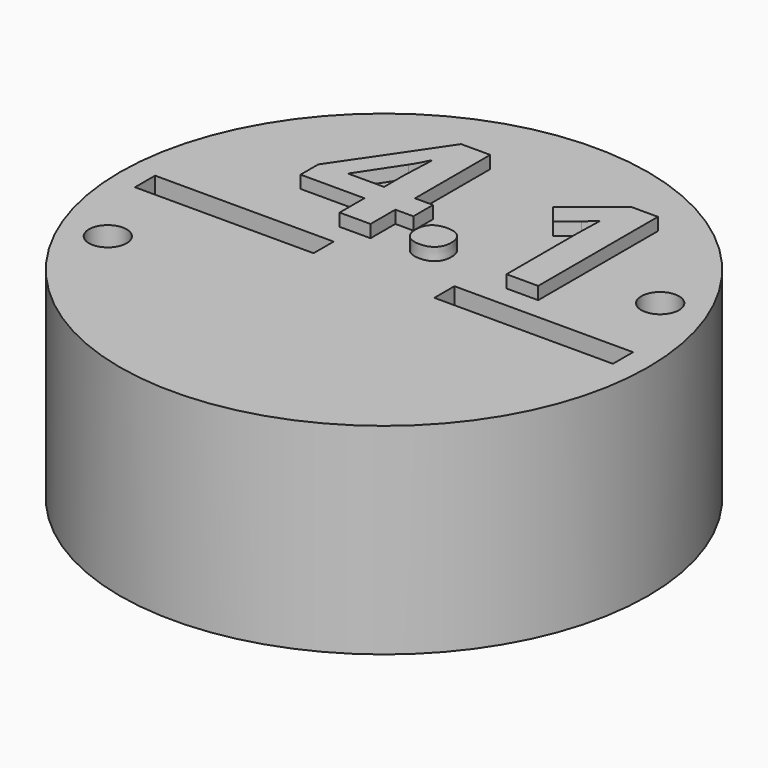
from build123d import *

# Parameters (mm, degrees)
F0_R          = 10.5
F1_DEPTH      = 8
F2_W          = 17.5
F2_H          = 1
F3_DEPTH      = 7
F5_DEPTH      = 17.5
F6_W          = 19
F6_H          = 1
F7_DEPTH      = 7
F9_DEPTH      = 19
F11_DEPTH     = 6.5
F12_R         = 0.75
F12_W         = 7.1
F12_H         = 1
F13_DEPTH     = 8
F14_TEXT_SIZE = 8.3333333333
F15_DEPTH     = 0.5


# Not quite as in the source:
# - Text() gives the source's letters only with a copy of the font that has no kerning and outlines rounded to 1/6400 em; it was checked with that copy


with BuildPart() as f1:
    # F0 (on Top) → F1 (new body)
    with BuildSketch(Plane.XY):
        Circle(F0_R)
    extrude(amount=-F1_DEPTH)

    # F2 (on face) → F3 (cut)
    with BuildSketch(Plane(origin=(0, 0, -8), x_dir=(1, 0, 0), z_dir=(0, 0, -1))):
        Rectangle(F2_W, F2_H)
    extrude(amount=-F3_DEPTH, mode=Mode.SUBTRACT)

    # F4 (on face) → F5 (cut)
    with BuildSketch(Plane(origin=(8.75, 0, 0), x_dir=(0, -1, 0), z_dir=(-1, 0, 0))):
        Polygon((-1.9558809371, -8), (1.9558809371, -8), (1.9558809371, -5), (0.5, -1), (-0.5, -1), (-1.9558809371, -5), align=None)
        Polygon((3, -1.5), (1.3, -1.5), (3, -6.1707116131), align=None)
        Polygon((-3, -6.1707116131), (-1.3, -1.5), (-3, -1.5), align=None)
    extrude(amount=F5_DEPTH, mode=Mode.SUBTRACT)

    # F6 (on face) → F7 (cut)
    with BuildSketch(Plane(origin=(0, 0, -8), x_dir=(1, 0, 0), z_dir=(0, 0, -1))):
        Rectangle(F6_W, F6_H)
    extrude(amount=-F7_DEPTH, mode=Mode.SUBTRACT)

    # F8 (on face) → F9 (cut)
    with BuildSketch(Plane(origin=(9.5, 0, 0), x_dir=(0, -1, 0), z_dir=(-1, 0, 0))):
        Polygon((1.0919107028, -8), (0, -5), (-1.0919107028, -8), align=None)
    extrude(amount=F9_DEPTH, mode=Mode.SUBTRACT)

    # F10 (on face) → F11 (cut)
    with BuildSketch(Plane(origin=(0, 0, -8), x_dir=(1, 0, 0), z_dir=(0, 0, -1))):
        with BuildLine():
            ThreePointArc((9.2870878105, 2.8), (0, 9.7), (-9.2870878105, 2.8))
            Line((-9.2870878105, 2.8), (9.2870878105, 2.8))
        make_face()
        with BuildLine():
            Line((9.3321359979, -2.8), (-9.3321359979, -2.8))
            ThreePointArc((-9.3321359979, -2.8), (0, -9.7431392417), (9.3321359979, -2.8))
        make_face()
    extrude(amount=-F11_DEPTH, mode=Mode.SUBTRACT)

    # F12 (on face) → F13 (cut)
    with BuildSketch(Plane(origin=(0, 0, -8), x_dir=(1, 0, 0), z_dir=(0, 0, -1))):
        with Locations((8.1, -3.6)):
            Circle(F12_R)
        with Locations((-8.1, 3.6)):
            Circle(F12_R)
        with Locations((5.95, 0)):
            Rectangle(F12_W, F12_H)
        with Locations((-5.95, 0)):
            Rectangle(F12_W, F12_H)
    extrude(amount=-F13_DEPTH, mode=Mode.SUBTRACT)

    # F14 (on face) → F15 (join)
    with BuildSketch(Plane.XY):
        with Locations((-5.5579427083, 1.3901121138)):
            Text('4.1', F14_TEXT_SIZE, font='Open Sans', font_style=FontStyle.BOLD, text_align=(TextAlign.LEFT, TextAlign.BOTTOM))
    extrude(amount=F15_DEPTH)


solid = f1.part
